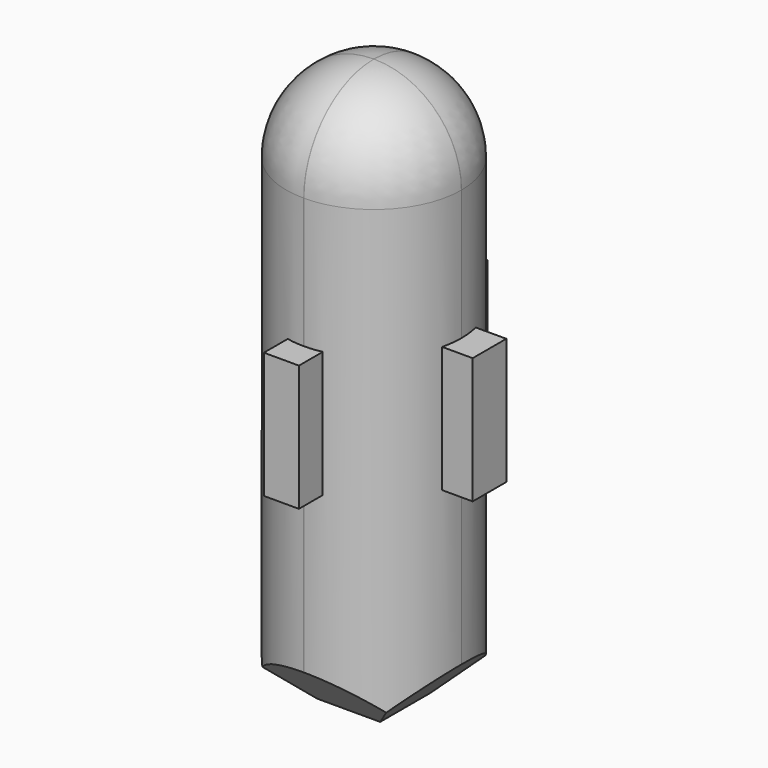
from build123d import *

# Parameters (mm, degrees)
F0_W          = 158.75
F0_H          = 508
F1_DEPTH      = 158.75
F3_W          = 38.1
F3_H          = 114.3
F4_DEPTH      = 25.4
F2_W          = 31.75
F2_H          = 114.3
F5_DEPTH      = 25.4
F6_R          = 78.74
F7_SIZE       = 50.8
F8_W          = 38.1
F8_H          = 114.3
F9_DEPTH      = 25.4
F10_T2_ANGLE  = 90
F10_T4_ANGLE  = 90
F10_T6_ANGLE  = 90
F10_T8_ANGLE  = 90
F10_T12_DEPTH = 655.32
F10_T17_DEPTH = 655.32
F10_T23_DEPTH = 655.32
F10_T28_DEPTH = 655.32
F10_T33_DEPTH = 655.32
F10_T38_DEPTH = 655.32
F10_T43_DEPTH = 655.32
F10_T48_DEPTH = 655.32
F10_T53_DEPTH = 655.32
F10_T58_DEPTH = 655.32
F10_T63_DEPTH = 655.32
F10_T69_DEPTH = 655.32


# Not quite as in the source:
# - a fillet or chamfer that OpenCascade refuses, or shapes differently, is made with other operations: its cross-section is extruded or revolved along the edge and cut away or added


with BuildPart() as f1:
    # F0 (on Front) → F1 (new body)
    with BuildSketch(Plane.XZ):
        Rectangle(F0_W, F0_H)
    extrude(amount=F1_DEPTH)

    # F3 (on face) → F4 (join)
    with BuildSketch(Plane.YZ.offset(79.375)):
        with Locations((-79.375, 0)):
            Rectangle(F3_W, F3_H)
    extrude(amount=F4_DEPTH)

    # F2 (on face) → F5 (join)
    with BuildSketch(Plane.XZ.offset(158.75)):
        Rectangle(F2_W, F2_H)
    extrude(amount=F5_DEPTH)

    # F6
    f6_edges = [f1.edges().sort_by_distance(p)[0] for p in [
        (79.375, -79.375, 254),
        (-79.375, -79.375, 254),
        (0, 0, 254),
        (0, -158.75, 254),
    ]]
    fillet(f6_edges, radius=F6_R)

    # F7
    f7_edges = [f1.edges().sort_by_distance(p)[0] for p in [
        (-79.375, -79.375, -254),
        (79.375, -79.375, -254),
        (0, 0, -254),
        (0, -158.75, -254),
    ]]
    chamfer(f7_edges, length=F7_SIZE)

    # F8 (on face) → F9 (join)
    with BuildSketch(Plane(origin=(0, 0, 0), x_dir=(-1, 0, 0), z_dir=(0, 1, 0))):
        Rectangle(F8_W, F8_H)
    extrude(amount=F9_DEPTH)

    # F10: fillet of radius 79.248 on 4 edges, made by hand

    # F10_s1 → F10_t2 (revolve, cut)
    with BuildSketch(Plane.YZ.offset(0.127)):
        with BuildLine():
            ThreePointArc((-80.01, 254), (-135.6875879506, 230.9375879506), (-158.75, 175.26))
            Line((-158.75, 175.26), (-158.75, 254))
            Line((-158.75, 254), (-80.01, 254))
        make_face()
    revolve(axis=Axis((0.127, -79.502, 254), (0, 0, 1)), revolution_arc=F10_T2_ANGLE, mode=Mode.SUBTRACT)

    # F10_s3 → F10_t4 (revolve, cut)
    with BuildSketch(Plane.YZ.offset(-0.127)):
        with BuildLine():
            ThreePointArc((-78.74, 254), (-23.0624120494, 230.9375879506), (0, 175.26))
            Line((0, 175.26), (0, 254))
            Line((0, 254), (-78.74, 254))
        make_face()
    revolve(axis=Axis((-0.127, -79.248, 254), (0, 0, 1)), revolution_arc=F10_T4_ANGLE, mode=Mode.SUBTRACT)

    # F10_s5 → F10_t6 (revolve, cut)
    with BuildSketch(Plane.XZ.offset(79.502)):
        with BuildLine():
            ThreePointArc((-0.635, 254), (-56.3125879506, 230.9375879506), (-79.375, 175.26))
            Line((-79.375, 175.26), (-79.375, 254))
            Line((-79.375, 254), (-0.635, 254))
        make_face()
    revolve(axis=Axis((-0.127, -79.502, 254), (0, 0, 1)), revolution_arc=F10_T6_ANGLE, mode=Mode.SUBTRACT)

    # F10_s7 → F10_t8 (revolve, cut)
    with BuildSketch(Plane.XZ.offset(79.248)):
        with BuildLine():
            ThreePointArc((0.635, 254), (56.3125879506, 230.9375879506), (79.375, 175.26))
            Line((79.375, 175.26), (79.375, 254))
            Line((79.375, 254), (0.635, 254))
        make_face()
    revolve(axis=Axis((0.127, -79.248, 254), (0, 0, 1)), revolution_arc=F10_T8_ANGLE, mode=Mode.SUBTRACT)


with BuildPart() as f10_tool10:
    # F10_s11 → F10_t12 (new body)
    with BuildSketch(Plane.XY.offset(-401.32)):
        with BuildLine():
            ThreePointArc((0.127, 0), (56.1637981955, -23.2112018045), (79.375, -79.248))
            Line((79.375, -79.248), (79.375, 0))
            Line((79.375, 0), (0.127, 0))
        make_face()
    extrude(amount=F10_T12_DEPTH)

    split(bisect_by=Plane.XY.offset(-57.15), keep=Keep.BOTTOM)


with BuildPart() as f1_1:
    add(f1.part)

    # F10_t9: cut F10_tool10
    add(f10_tool10.part, mode=Mode.SUBTRACT)


with BuildPart() as f10_tool15:
    # F10_s16 → F10_t17 (new body)
    with BuildSketch(Plane.XY.offset(-401.32)):
        with BuildLine():
            ThreePointArc((0.127, 0), (56.1637981955, -23.2112018045), (79.375, -79.248))
            Line((79.375, -79.248), (79.375, 0))
            Line((79.375, 0), (0.127, 0))
        make_face()
    extrude(amount=F10_T17_DEPTH)

    split(bisect_by=Plane.YZ.offset(19.05), keep=Keep.TOP)

    split(bisect_by=Plane.XZ.offset(60.325), keep=Keep.BOTTOM)


with BuildPart() as f1_2:
    add(f1_1.part)

    # F10_t14: cut F10_tool15
    add(f10_tool15.part, mode=Mode.SUBTRACT)


with BuildPart() as f10_tool21:
    # F10_s22 → F10_t23 (new body)
    with BuildSketch(Plane.XY.offset(-401.32)):
        with BuildLine():
            ThreePointArc((0.127, 0), (56.1637981955, -23.2112018045), (79.375, -79.248))
            Line((79.375, -79.248), (79.375, 0))
            Line((79.375, 0), (0.127, 0))
        make_face()
    extrude(amount=F10_T23_DEPTH)

    split(bisect_by=Plane.XY.offset(57.15), keep=Keep.TOP)


with BuildPart() as f1_3:
    add(f1_2.part)

    # F10_t20: cut F10_tool21
    add(f10_tool21.part, mode=Mode.SUBTRACT)


with BuildPart() as f10_tool26:
    # F10_s27 → F10_t28 (new body)
    with BuildSketch(Plane.XY.offset(254)):
        with BuildLine():
            ThreePointArc((-79.375, -79.502), (-56.1637981955, -135.5387981955), (-0.127, -158.75))
            Line((-0.127, -158.75), (-79.375, -158.75))
            Line((-79.375, -158.75), (-79.375, -79.502))
        make_face()
    extrude(amount=-F10_T28_DEPTH)

    split(bisect_by=Plane.XY.offset(57.15), keep=Keep.TOP)


with BuildPart() as f1_4:
    add(f1_3.part)

    # F10_t25: cut F10_tool26
    add(f10_tool26.part, mode=Mode.SUBTRACT)


with BuildPart() as f10_tool31:
    # F10_s32 → F10_t33 (new body)
    with BuildSketch(Plane.XY.offset(254)):
        with BuildLine():
            ThreePointArc((-79.375, -79.502), (-56.1637981955, -135.5387981955), (-0.127, -158.75))
            Line((-0.127, -158.75), (-79.375, -158.75))
            Line((-79.375, -158.75), (-79.375, -79.502))
        make_face()
    extrude(amount=-F10_T33_DEPTH)

    split(bisect_by=Plane.YZ.offset(-15.875), keep=Keep.BOTTOM)


with BuildPart() as f1_5:
    add(f1_4.part)

    # F10_t30: cut F10_tool31
    add(f10_tool31.part, mode=Mode.SUBTRACT)


with BuildPart() as f10_tool36:
    # F10_s37 → F10_t38 (new body)
    with BuildSketch(Plane.XY.offset(254)):
        with BuildLine():
            ThreePointArc((-79.375, -79.502), (-56.1637981955, -135.5387981955), (-0.127, -158.75))
            Line((-0.127, -158.75), (-79.375, -158.75))
            Line((-79.375, -158.75), (-79.375, -79.502))
        make_face()
    extrude(amount=-F10_T38_DEPTH)

    split(bisect_by=Plane.XY.offset(-57.15), keep=Keep.BOTTOM)


with BuildPart() as f1_6:
    add(f1_5.part)

    # F10_t35: cut F10_tool36
    add(f10_tool36.part, mode=Mode.SUBTRACT)


with BuildPart() as f10_tool41:
    # F10_s42 → F10_t43 (new body)
    with BuildSketch(Plane.XY.offset(254)):
        with BuildLine():
            ThreePointArc((-79.375, -79.248), (-56.1637981955, -23.2112018045), (-0.127, 0))
            Line((-0.127, 0), (-79.375, 0))
            Line((-79.375, 0), (-79.375, -79.248))
        make_face()
    extrude(amount=-F10_T43_DEPTH)

    split(bisect_by=Plane.XY.offset(57.15), keep=Keep.TOP)


with BuildPart() as f1_7:
    add(f1_6.part)

    # F10_t40: cut F10_tool41
    add(f10_tool41.part, mode=Mode.SUBTRACT)


with BuildPart() as f10_tool46:
    # F10_s47 → F10_t48 (new body)
    with BuildSketch(Plane.XY.offset(254)):
        with BuildLine():
            ThreePointArc((-79.375, -79.248), (-56.1637981955, -23.2112018045), (-0.127, 0))
            Line((-0.127, 0), (-79.375, 0))
            Line((-79.375, 0), (-79.375, -79.248))
        make_face()
    extrude(amount=-F10_T48_DEPTH)

    split(bisect_by=Plane.YZ.offset(-19.05), keep=Keep.BOTTOM)


with BuildPart() as f1_8:
    add(f1_7.part)

    # F10_t45: cut F10_tool46
    add(f10_tool46.part, mode=Mode.SUBTRACT)


with BuildPart() as f10_tool51:
    # F10_s52 → F10_t53 (new body)
    with BuildSketch(Plane.XY.offset(254)):
        with BuildLine():
            ThreePointArc((-79.375, -79.248), (-56.1637981955, -23.2112018045), (-0.127, 0))
            Line((-0.127, 0), (-79.375, 0))
            Line((-79.375, 0), (-79.375, -79.248))
        make_face()
    extrude(amount=-F10_T53_DEPTH)

    split(bisect_by=Plane.XY.offset(-57.15), keep=Keep.BOTTOM)


with BuildPart() as f1_9:
    add(f1_8.part)

    # F10_t50: cut F10_tool51
    add(f10_tool51.part, mode=Mode.SUBTRACT)


with BuildPart() as f10_tool56:
    # F10_s57 → F10_t58 (new body)
    with BuildSketch(Plane.XY.offset(-401.32)):
        with BuildLine():
            ThreePointArc((0.127, -158.75), (56.1637981955, -135.5387981955), (79.375, -79.502))
            Line((79.375, -79.502), (79.375, -158.75))
            Line((79.375, -158.75), (0.127, -158.75))
        make_face()
    extrude(amount=F10_T58_DEPTH)

    split(bisect_by=Plane.XY.offset(-57.15), keep=Keep.BOTTOM)


with BuildPart() as f1_10:
    add(f1_9.part)

    # F10_t55: cut F10_tool56
    add(f10_tool56.part, mode=Mode.SUBTRACT)


with BuildPart() as f10_tool61:
    # F10_s62 → F10_t63 (new body)
    with BuildSketch(Plane.XY.offset(-401.32)):
        with BuildLine():
            ThreePointArc((0.127, -158.75), (56.1637981955, -135.5387981955), (79.375, -79.502))
            Line((79.375, -79.502), (79.375, -158.75))
            Line((79.375, -158.75), (0.127, -158.75))
        make_face()
    extrude(amount=F10_T63_DEPTH)

    split(bisect_by=Plane.YZ.offset(15.875), keep=Keep.TOP)

    split(bisect_by=Plane.XZ.offset(98.425), keep=Keep.TOP)


with BuildPart() as f1_11:
    add(f1_10.part)

    # F10_t60: cut F10_tool61
    add(f10_tool61.part, mode=Mode.SUBTRACT)


with BuildPart() as f10_tool67:
    # F10_s68 → F10_t69 (new body)
    with BuildSketch(Plane.XY.offset(-401.32)):
        with BuildLine():
            ThreePointArc((0.127, -158.75), (56.1637981955, -135.5387981955), (79.375, -79.502))
            Line((79.375, -79.502), (79.375, -158.75))
            Line((79.375, -158.75), (0.127, -158.75))
        make_face()
    extrude(amount=F10_T69_DEPTH)

    split(bisect_by=Plane.XY.offset(57.15), keep=Keep.TOP)


with BuildPart() as f1_12:
    add(f1_11.part)

    # F10_t66: cut F10_tool67
    add(f10_tool67.part, mode=Mode.SUBTRACT)


solid = f1_12.part
